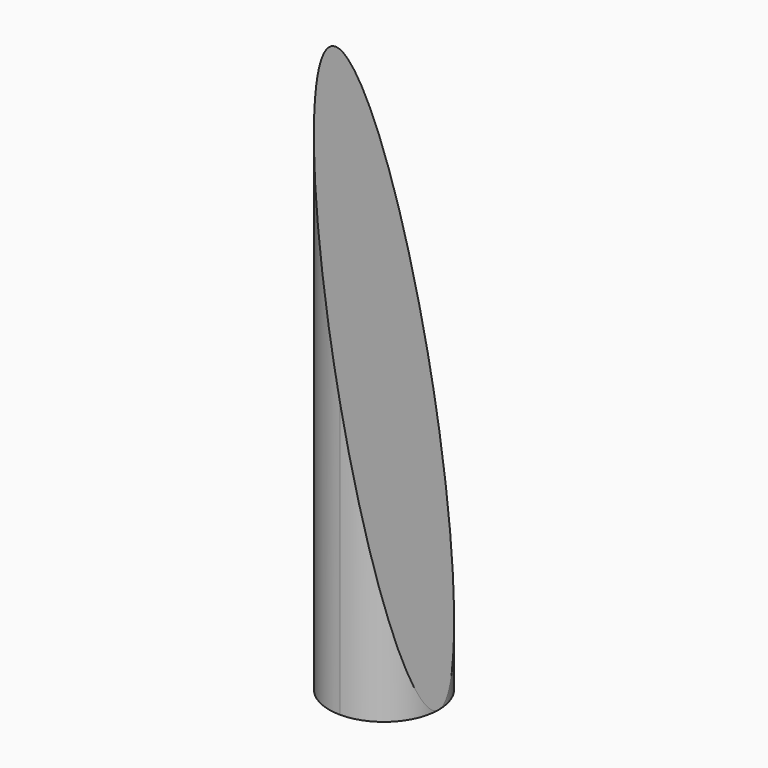
from build123d import *

# Parameters (mm, degrees)
F1_DEPTH = 25.4
F3_DEPTH = 254


with BuildPart() as f1:
    # F0 (on Front) → F1 (new body, symmetric)
    with BuildSketch(Plane.XZ):
        Polygon((-25.4, 254), (-25.4, 0), (25.4, 0), align=None)
    extrude(amount=F1_DEPTH, both=True)

    # F2 (on face) → F3 (cut)
    with BuildSketch(Plane(origin=(0, 0, 0), x_dir=(1, 0, 0), z_dir=(0, 0, -1))):
        with BuildLine():
            ThreePointArc((4.89e-08, 25.4), (17.9605122594, 17.9605122249), (25.4, 0))
            Line((25.4, 0), (25.4, 25.4))
            Line((25.4, 25.4), (4.89e-08, 25.4))
        make_face()
        with BuildLine():
            Line((25.4, -25.4), (25.4, 0))
            ThreePointArc((25.4, 0), (17.9605122528, -17.9605122315), (3.01e-08, -25.4))
            Line((3.01e-08, -25.4), (25.4, -25.4))
        make_face()
        with BuildLine():
            Line((-25.4, -25.4), (3.01e-08, -25.4))
            ThreePointArc((3.01e-08, -25.4), (-17.9605122437, -17.9605122406), (-25.4, 3.44e-08))
            Line((-25.4, 3.44e-08), (-25.4, -25.4))
        make_face()
        with BuildLine():
            ThreePointArc((-25.4, 3.44e-08), (-17.9605122127, 17.9605122716), (4.89e-08, 25.4))
            Line((4.89e-08, 25.4), (-25.4, 25.4))
            Line((-25.4, 25.4), (-25.4, 3.44e-08))
        make_face()
    extrude(amount=-F3_DEPTH, mode=Mode.SUBTRACT)


solid = f1.part
